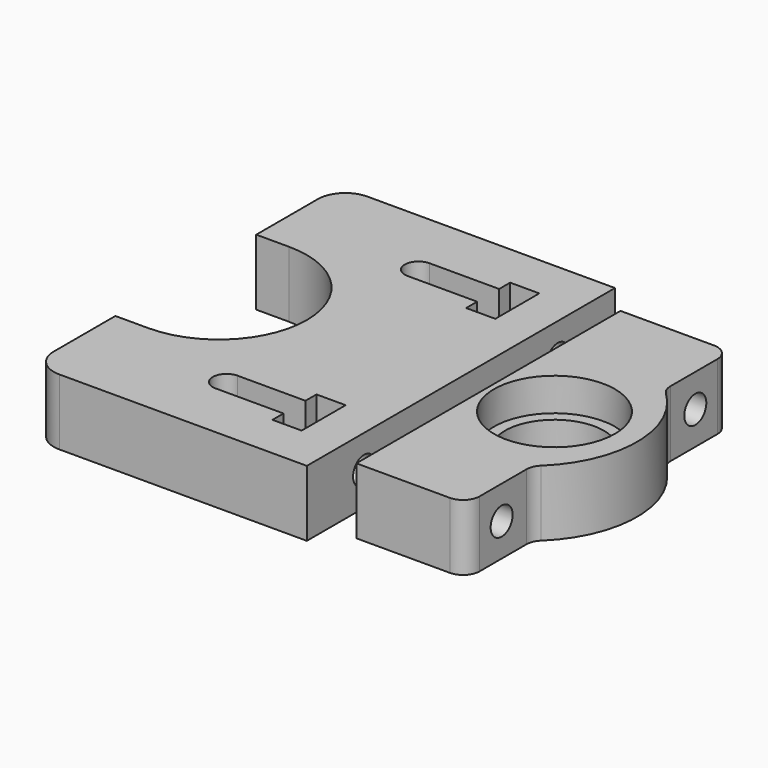
from build123d import *

# Parameters (mm, degrees)
F1_DEPTH  = 12
F2_R      = 2.5
F3_DEPTH  = 15
F4_R      = 5
F5_R      = 11
F6_DEPTH  = 12
F5_R_2    = 9
F7_DEPTH  = 6
F8_R      = 3
F6_FACE_W = 10.6598653616
F6_FACE_H = 12
F9_DEPTH  = 25


# Not quite as in the source:
# - a feature names something its author has since deleted; it is built from what else it names


with BuildPart() as f1:
    # F0 (on Top) → F1 (new body)
    with BuildSketch(Plane.XY):
        with BuildLine():
            Line((6.2480168641, -35), (6.2480168641, 0))
            Line((6.2480168641, 0), (6.2480168641, 35))
            Line((6.2480168641, 35), (-43.7519831359, 35))
            Line((-43.7519831359, 35), (-43.7519831359, 16))
            Line((-43.7519831359, 16), (-37.7519831359, 16))
            ThreePointArc((-37.7519831359, 16), (-21.7519831359, 0), (-37.7519831359, -16))
            Line((-37.7519831359, -16), (-43.7519831359, -16))
            Line((-43.7519831359, -16), (-43.7519831359, -35))
            Line((-43.7519831359, -35), (6.2480168641, -35))
        make_face()
        with BuildLine():
            ThreePointArc((-18.7519831359, -24.5), (-21.2519831359, -22), (-18.7519831359, -19.5))
            Line((-18.7519831359, -19.5), (-6.4019831359, -19.5))
            Line((-6.4019831359, -19.5), (-6.4019831359, -17))
            Line((-6.4019831359, -17), (-1.1019831359, -17))
            Line((-1.1019831359, -17), (-1.1019831359, -27))
            Line((-1.1019831359, -27), (-6.4019831359, -27))
            Line((-6.4019831359, -27), (-6.4019831359, -24.5))
            Line((-6.4019831359, -24.5), (-18.7519831359, -24.5))
        make_face(mode=Mode.SUBTRACT)
        with BuildLine():
            ThreePointArc((-19.0519835278, 19.4999995902), (-21.5519835278, 21.9999995902), (-19.0519835278, 24.4999995902))
            Line((-19.0519835278, 24.4999995902), (-6.4019831359, 24.500000484))
            Line((-6.4019831359, 24.500000484), (-6.4019831359, 27))
            Line((-6.4019831359, 27), (-1.1019831359, 27))
            Line((-1.1019831359, 27), (-1.1019831359, 17))
            Line((-1.1019831359, 17), (-6.4019831359, 17))
            Line((-6.4019831359, 17), (-6.4019831359, 19.500000484))
            Line((-6.4019831359, 19.500000484), (-19.0519835278, 19.4999995902))
        make_face(mode=Mode.SUBTRACT)
    extrude(amount=F1_DEPTH)

    # F2 (on face) → F3 (cut)
    with BuildSketch(Plane.YZ.offset(6.2480168641)):
        with Locations((-22, 6)):
            Circle(F2_R)
        with Locations((22, 6)):
            Circle(F2_R)
    extrude(amount=-F3_DEPTH, mode=Mode.SUBTRACT)

    # F4
    f4_edges = [f1.edges().sort_by_distance(p)[0] for p in [
        (-43.751983, 35, 6),
        (-43.751983, -35, 6),
    ]]
    fillet(f4_edges, radius=F4_R)


with BuildPart() as f6:
    # F5 (on Top) → F6 (new body)
    with BuildSketch(Plane.XY):
        with BuildLine():
            Line((31.2480168641, 30), (11.2480168641, 30))
            Line((11.2480168641, 30), (11.2480168641, -30))
            Line((11.2480168641, -30), (31.2480168641, -30))
            Line((31.2480168641, -30), (31.2480168641, -15))
            ThreePointArc((31.2480168641, -15), (38.2480168641, 0), (31.2480168641, 15))
            Line((31.2480168641, 15), (31.2480168641, 30))
        make_face()
        with Locations((23.2480168641, 0)):
            Circle(F5_R, mode=Mode.SUBTRACT)
    extrude(amount=F6_DEPTH)

    # F5 (on Top) → F7 (join)
    with BuildSketch(Plane.XY):
        with Locations((23.2480168641, 0)):
            Circle(F5_R)
        with Locations((23.2480168641, 0)):
            Circle(F5_R_2, mode=Mode.SUBTRACT)
    extrude(amount=F7_DEPTH)

    # F8
    f8_edges = [f6.edges().sort_by_distance(p)[0] for p in [
        (31.248017, 30, 6),
        (31.248017, -30, 6),
        (31.248017, 15, 6),
        (31.248017, -15, 6),
    ]]
    fillet(f8_edges, radius=F8_R)

    # F2 (on face) + F6_face (on face) → F9 (cut)
    with BuildSketch(Plane.YZ.offset(6.2480168641)):
        with Locations((-22, 6)):
            Circle(F2_R)
        with Locations((22, 6)):
            Circle(F2_R)
    with BuildSketch(Plane(origin=(31.2480168641, 21.6700673192, 6), x_dir=(0, 1, 0), z_dir=(1, 0, 0))):
        Rectangle(F6_FACE_W, F6_FACE_H)
    extrude(amount=F9_DEPTH, mode=Mode.SUBTRACT)


solid = Compound([f1.part, f6.part])
